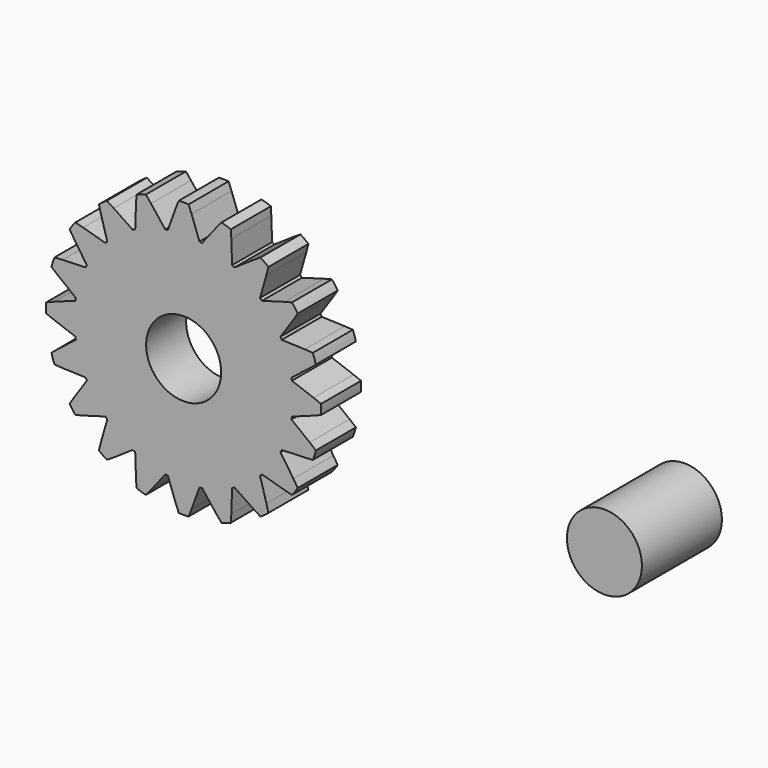
from build123d import *

# Parameters (mm, degrees)
F1_R     = 0.75
F2_DEPTH = 1
F3_COUNT = 20
F3_ANGLE = 342
F4_R     = 0.75
F5_DEPTH = 2


# Not quite as in the source:
# - a feature names something its author has since deleted; it is built from what else it names


with BuildPart() as f2:
    # F1 (on Front) → F2 (new body)
    with BuildSketch(Plane.XZ):
        with BuildLine():
            Line((-0.1578473268, 2.598060965), (-0.3156097094, 2.1646123813))
            ThreePointArc((-0.3156097094, 2.1646123813), (0, -2.1875), (0.3156097094, 2.1646123813))
            Line((0.3156097094, 2.1646123813), (0.1578473268, 2.598060965))
            add(Edge.make_bspline(
                [(0.1578473268, 2.598060965), (0.1484563179, 2.6250683902), (0.1308720869, 2.6755639646), (0.10907726, 2.7242678255), (0.0982551486, 2.7482441532)],
                knots=[0, 0, 0, 0, 0.5054135762, 1, 1, 1, 1], degree=3))
            ThreePointArc((0.0982551486, 2.7482441532), (0, 2.7520262365), (-0.0982551486, 2.7482441532))
            add(Edge.make_bspline(
                [(-0.1578473268, 2.598060965), (-0.1484563179, 2.6250683902), (-0.1308720869, 2.6755639646), (-0.10907726, 2.7242678255), (-0.0982551486, 2.7482441532)],
                knots=[0, 0, 0, 0, 0.5054135762, 1, 1, 1, 1], degree=3))
        make_face()
        Circle(F1_R, mode=Mode.SUBTRACT)
    extrude(amount=F2_DEPTH)

    # F3: F2 ×20 about axis
    f3_axis = Axis((0, 0, 0), (0, -1, 0))


with BuildPart() as f2_1:
    add(f2.part)
    for i in range(1, F3_COUNT):
        add(f2.part.rotate(f3_axis, i * F3_ANGLE / (F3_COUNT - 1)))


with BuildPart() as f5:
    # F4 (on Front) → F5 (new body)
    with BuildSketch(Plane.XZ):
        with Locations((9.2156029012, 0)):
            Circle(F4_R)
    extrude(amount=F5_DEPTH)


solid = Compound([f2_1.part, f5.part])
